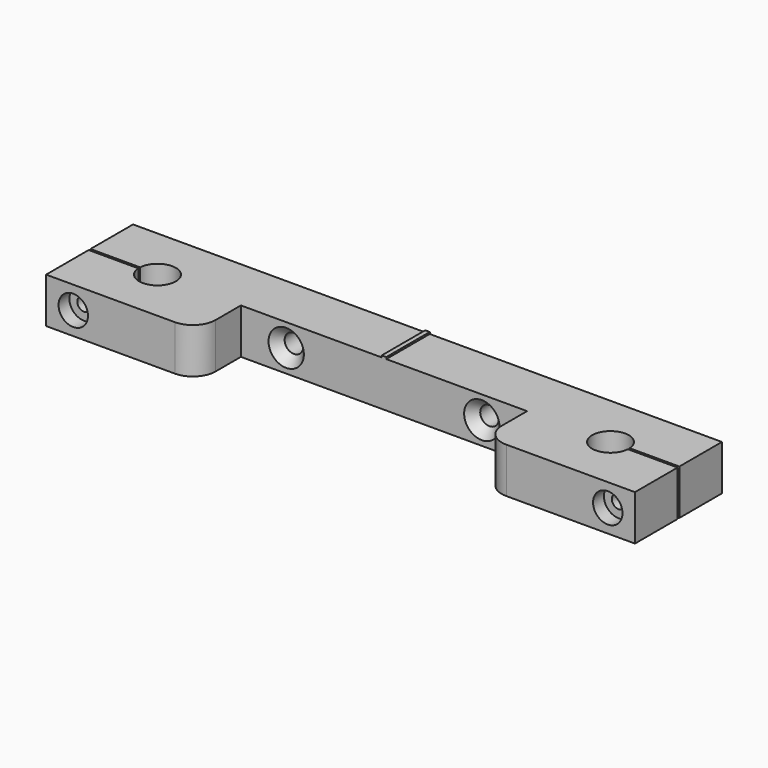
from build123d import *

# Parameters (mm, degrees)
F0_R            = 4.05
F1_DEPTH        = 10
F2_R            = 5
F4_D            = 4.1000000042
F4_CSINK_D      = 7.7978
F4_CSINK_ANGLE  = 82
F5_W            = 1
F5_H            = 12
F6_DEPTH        = 0.4
F8_DEPTH        = 25
F10_D           = 3
F10_CBORE_D     = 6.5
F10_CBORE_DEPTH = 3


with BuildPart() as f1:
    # F0 (on Top) → F1 (new body)
    with BuildSketch(Plane.XY):
        Polygon((67.5994434953, -8.2149432153), (-62.4005565047, -8.2149432153), (-62.4005565047, -32.2149432153), (-28.9914757013, -32.2149432153), (-28.9914757013, -20.2149432153), (34.1903626919, -20.2149432153), (34.1903626919, -32.2149432153), (67.5994434953, -32.2149432153), align=None)
        with Locations((-47.4005565047, -20.2149432153)):
            Circle(F0_R, mode=Mode.SUBTRACT)
        with Locations((52.5994434953, -20.2149432153)):
            Circle(F0_R, mode=Mode.SUBTRACT)
    extrude(amount=F1_DEPTH)

    # F2
    f2_edges = [f1.edges().sort_by_distance(p)[0] for p in [
        (34.190363, -32.214943, 5),
        (-28.991476, -32.214943, 5),
    ]]
    fillet(f2_edges, radius=F2_R)

    # F4 (through all)
    with Locations(Plane.XZ.offset(20.2149432153)):
        with Locations((-18.9914757013, 5), (24.1903626919, 5)):
            CounterSinkHole(F4_D / 2, F4_CSINK_D / 2, counter_sink_angle=F4_CSINK_ANGLE)

    # F5 (on face) → F6 (join)
    with BuildSketch(Plane.XY.offset(10)):
        with Locations((2.5994434953, -14.2149432153)):
            Rectangle(F5_W, F5_H)
    extrude(amount=F6_DEPTH)

    # F7 (on face) → F8 (cut)
    with BuildSketch(Plane.XY.offset(10)):
        with BuildLine():
            ThreePointArc((56.6417200816, -19.9649432153), (56.6475121814, -20.0898835784), (56.6494434953, -20.2149432153))
            ThreePointArc((56.6494434953, -20.2149432153), (56.6475121814, -20.3400028521), (56.6417200816, -20.4649432153))
            Line((56.6417200816, -20.4649432153), (67.5994434953, -20.4649432153))
            Line((67.5994434953, -20.4649432153), (67.5994434953, -19.9649432153))
            Line((67.5994434953, -19.9649432153), (56.6417200816, -19.9649432153))
        make_face()
        with BuildLine():
            Line((-51.442833091, -19.9649432153), (-62.4005565047, -19.9649432153))
            Line((-62.4005565047, -19.9649432153), (-62.4005565047, -20.4649432153))
            Line((-62.4005565047, -20.4649432153), (-51.442833091, -20.4649432153))
            ThreePointArc((-51.442833091, -20.4649432153), (-51.4505565047, -20.2149432153), (-51.442833091, -19.9649432153))
        make_face()
        with BuildLine():
            Line((-51.442833091, -20.4649432153), (-51.442833091, -19.9649432153))
            ThreePointArc((-51.442833091, -19.9649432153), (-51.4505565047, -20.2149432153), (-51.442833091, -20.4649432153))
        make_face()
        with BuildLine():
            ThreePointArc((56.6417200816, -20.4649432153), (56.6475121814, -20.3400028521), (56.6494434953, -20.2149432153))
            ThreePointArc((56.6494434953, -20.2149432153), (56.6475121814, -20.0898835784), (56.6417200816, -19.9649432153))
            Line((56.6417200816, -19.9649432153), (56.6417200816, -20.4649432153))
        make_face()
    extrude(amount=-F8_DEPTH, mode=Mode.SUBTRACT)

    # F10 (through all)
    with Locations(Plane.XZ.offset(32.2149432153)):
        with Locations((61.5994434953, 5), (-56.4005565047, 5)):
            CounterBoreHole(F10_D / 2, F10_CBORE_D / 2, F10_CBORE_DEPTH)


solid = f1.part
